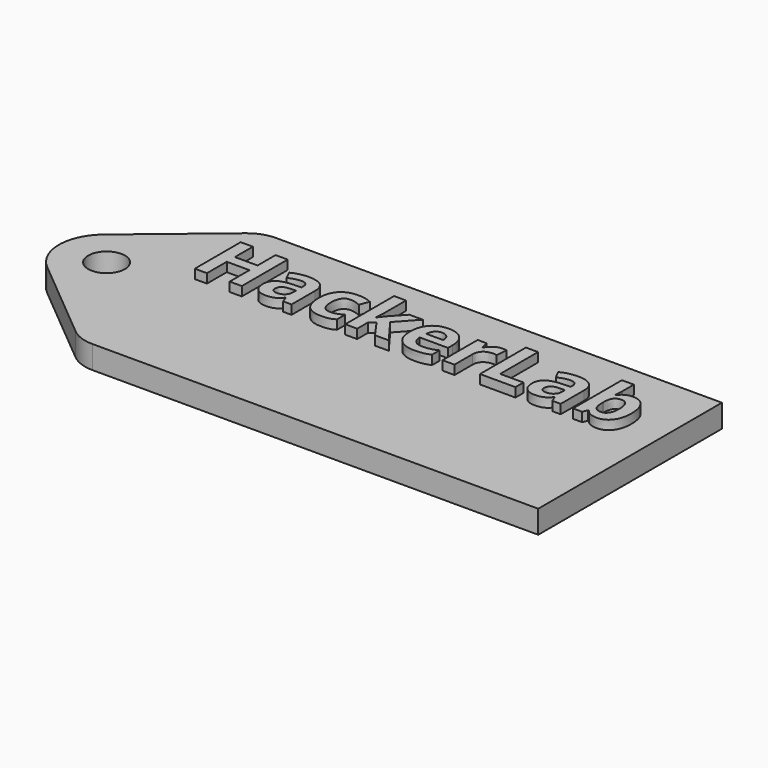
from build123d import *

# Parameters (mm, degrees)
F0_W         = 63.5
F0_H         = 31.75
F0_R         = 2.54
F1_DEPTH     = 3.175
F2_R         = 5.08
F3_TEXT_SIZE = 11.1148094268
F4_DEPTH     = 1.27


# Not quite as in the source:
# - Text() gives the source's letters only with a copy of the font that has no kerning and outlines rounded to 1/6400 em; it was checked with that copy


with BuildPart() as f1:
    # F0 (on Top) → F1 (new body)
    with BuildSketch(Plane.XY):
        with Locations((31.75, 15.875)):
            Rectangle(F0_W, F0_H)
        with BuildLine():
            Line((-13.1961538495, 10.9967948746), (0, 0))
            Line((0, 0), (0, 31.75))
            Line((0, 31.75), (-13.1961538495, 20.7532051254))
            ThreePointArc((-13.1961538495, 20.7532051254), (-15.4809829116, 15.875), (-13.1961538495, 10.9967948746))
        make_face()
        with Locations((-8.89, 15.875)):
            Circle(F0_R, mode=Mode.SUBTRACT)
    extrude(amount=F1_DEPTH)

    # F2
    f2_edges = [f1.edges().sort_by_distance(p)[0] for p in [
        (0, 31.75, 1.5875),
        (0, 0, 1.5875),
    ]]
    fillet(f2_edges, radius=F2_R)

    # F3 (on face) → F4 (join)
    with BuildSketch(Plane.XY.offset(3.175)):
        with Locations((0, 18.7556097325)):
            Text('HackerLab', F3_TEXT_SIZE, font='Open Sans', font_style=FontStyle.BOLD, text_align=(TextAlign.LEFT, TextAlign.BOTTOM))
    extrude(amount=F4_DEPTH)


solid = f1.part
